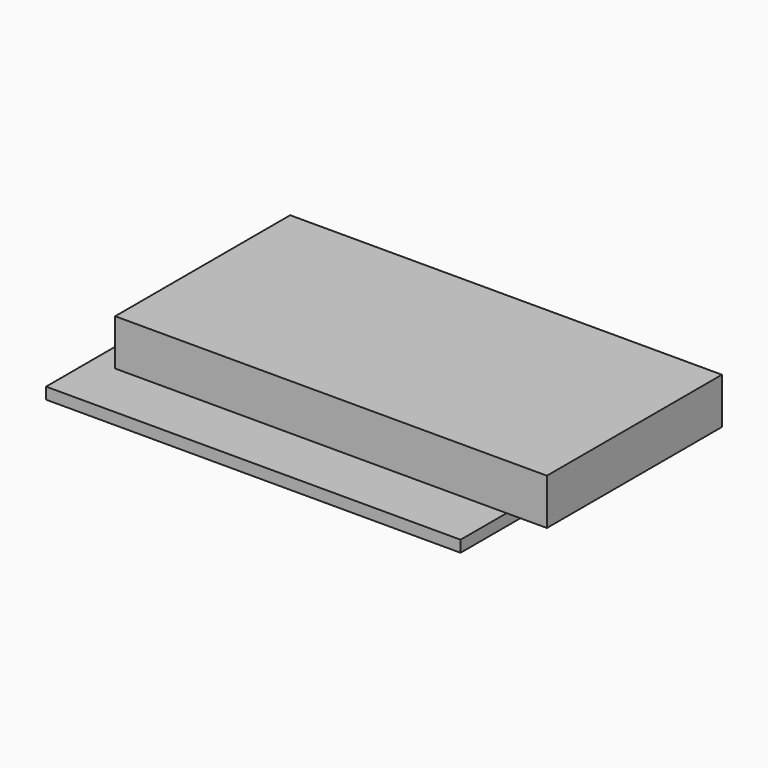
from build123d import *

# Parameters (mm, degrees)
F0_W      = 1828.8
F0_H      = 1219.2
F1_DEPTH  = 50.8
F6_DEPTH  = 25.4
F8_DEPTH  = 25.4
F9_W      = 1905
F9_H      = 965.2
F10_DEPTH = 203.2


# Not quite as in the source:
# - a feature of the source that left no trace in its solid (it failed there, or was rolled back) is left out


with BuildPart() as f1:
    # F0 (on Top) → F1 (new body)
    with BuildSketch(Plane.XY):
        with Locations((914.4, 609.6)):
            Rectangle(F0_W, F0_H)
    extrude(amount=F1_DEPTH)

    # F5 (on face) → F6 (cut)
    with BuildSketch(Plane.XZ):
        with BuildLine():
            Line((1254.4775691986, 50.8), (1711.6775691986, 50.8))
            ThreePointArc((1711.6775691986, 50.8), (1783.5196181672, 80.5579510314), (1813.2775691986, 152.4))
            Line((1813.2775691986, 152.4), (1813.2775691986, 863.6))
            ThreePointArc((1813.2775691986, 863.6), (1783.5196181672, 935.4420489686), (1711.6775691986, 965.2))
            Line((1711.6775691986, 965.2), (1254.4775691986, 965.2))
            ThreePointArc((1254.4775691986, 965.2), (1182.6355202301, 935.4420489686), (1152.8775691986, 863.6))
            Line((1152.8775691986, 863.6), (1152.8775691986, 152.4))
            ThreePointArc((1152.8775691986, 152.4), (1182.6355202301, 80.5579510314), (1254.4775691986, 50.8))
        make_face()
    extrude(amount=-F6_DEPTH, mode=Mode.SUBTRACT)

    # F7 (on face) → F8 (cut)
    with BuildSketch(Plane(origin=(0, 1219.2, 0), x_dir=(-1, 0, 0), z_dir=(0, 1, 0))):
        with BuildLine():
            Line((-1854.2, 736.6), (-2133.6, 736.6))
            ThreePointArc((-2133.6, 736.6), (-2169.5210244843, 721.7210244843), (-2184.4, 685.8))
            Line((-2184.4, 685.8), (-2184.4, 558.8))
            ThreePointArc((-2184.4, 558.8), (-2169.5210244843, 522.8789755157), (-2133.6, 508))
            Line((-2133.6, 508), (-1854.2, 508))
            ThreePointArc((-1854.2, 508), (-1818.2789755157, 522.8789755157), (-1803.4, 558.8))
            Line((-1803.4, 558.8), (-1803.4, 685.8))
            ThreePointArc((-1803.4, 685.8), (-1818.2789755157, 721.7210244843), (-1854.2, 736.6))
        make_face()
    extrude(amount=-F8_DEPTH, mode=Mode.SUBTRACT)


with BuildPart() as f10:
    # F9 (on face) → F10 (new body)
    with BuildSketch(Plane.XY.offset(50.8)):
        with Locations((1054.1, 736.6)):
            Rectangle(F9_W, F9_H)
    extrude(amount=F10_DEPTH)


solid = Compound([f1.part, f10.part])
